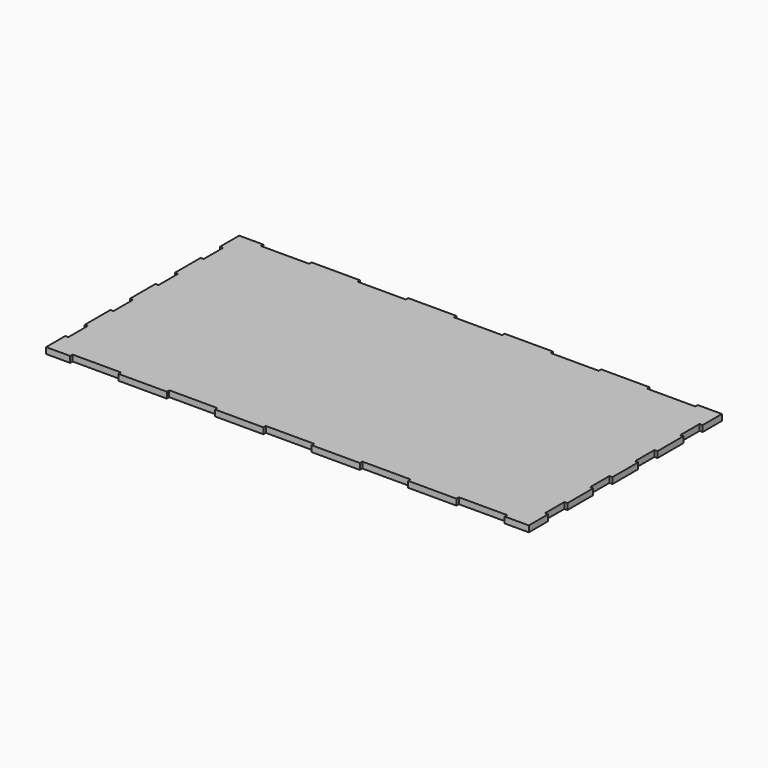
from build123d import *

# Parameters (mm, degrees)
F0_W     = 500
F0_H     = 250
F1_DEPTH = 6.35
F2_W     = 50
F2_H     = 3.175
F2_W_2   = 3.175
F2_H_2   = 25
F3_DEPTH = 6.351


# Not quite as in the source:
# - a length typed as a fraction of an inch, garbled in the dataset ("3 / 203.2 mm" for 3/8 in), is restored


with BuildPart() as f1:
    # F0 (on Top) → F1 (new body)
    with BuildSketch(Plane.XY):
        Rectangle(F0_W, F0_H)
    extrude(amount=F1_DEPTH)

    # F2 (on face) → F3 (cut, through all)
    with BuildSketch(Plane.XY.offset(6.35)):
        with Locations((-200, 123.4125)):
            Rectangle(F2_W, F2_H)
        with Locations((-200, -123.4125)):
            Rectangle(F2_W, F2_H)
        with Locations((-100, 123.4125)):
            Rectangle(F2_W, F2_H)
        with Locations((-100, -123.4125)):
            Rectangle(F2_W, F2_H)
        with Locations((0, 123.4125)):
            Rectangle(F2_W, F2_H)
        with Locations((0, -123.4125)):
            Rectangle(F2_W, F2_H)
        with Locations((100, 123.4125)):
            Rectangle(F2_W, F2_H)
        with Locations((100, -123.4125)):
            Rectangle(F2_W, F2_H)
        with Locations((200, 123.4125)):
            Rectangle(F2_W, F2_H)
        with Locations((200, -123.4125)):
            Rectangle(F2_W, F2_H)
        with Locations((248.4125, 87.5)):
            Rectangle(F2_W_2, F2_H_2)
        with Locations((248.4125, 29.1666666667)):
            Rectangle(F2_W_2, F2_H_2)
        with Locations((248.4125, -29.1666666667)):
            Rectangle(F2_W_2, F2_H_2)
        with Locations((248.4125, -87.5)):
            Rectangle(F2_W_2, F2_H_2)
        with Locations((-248.4125, -87.5)):
            Rectangle(F2_W_2, F2_H_2)
        with Locations((-248.4125, 29.1666666667)):
            Rectangle(F2_W_2, F2_H_2)
        with Locations((-248.4125, -29.1666666667)):
            Rectangle(F2_W_2, F2_H_2)
        with Locations((-248.4125, 87.5)):
            Rectangle(F2_W_2, F2_H_2)
    extrude(amount=-F3_DEPTH, mode=Mode.SUBTRACT)


solid = f1.part
